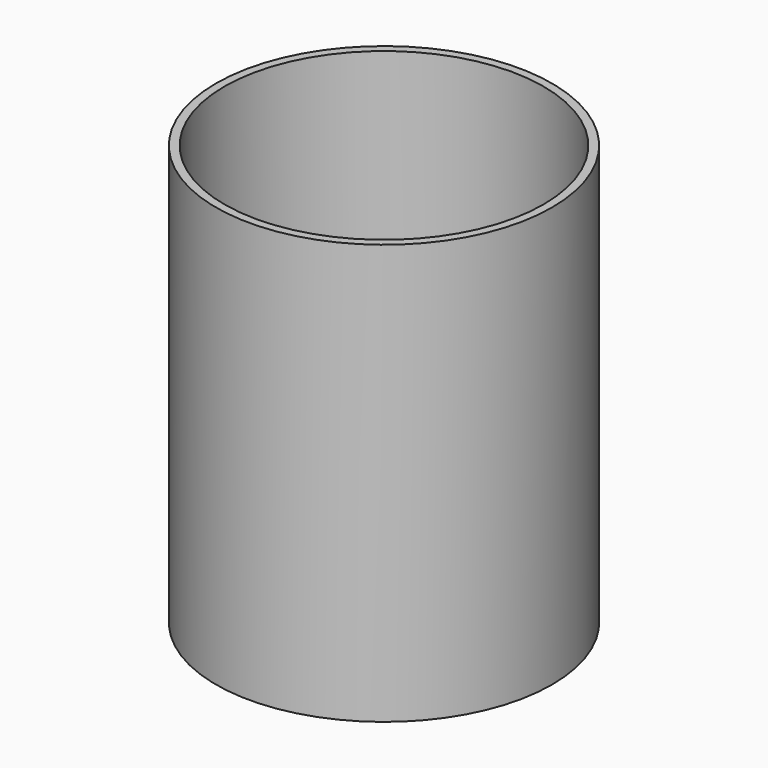
from build123d import *

# Parameters (mm, degrees)
F0_R     = 50.8
F1_DEPTH = 63.5
F2_T     = -2.54


# Not quite as in the source:
# - the program builds the solid bodies; features that only make, move or delete a surface that nothing else refers to are left out


with BuildPart() as f1:
    # F0 (on Top) → F1 (new body, symmetric)
    with BuildSketch(Plane.XY):
        Circle(F0_R)
    extrude(amount=F1_DEPTH, both=True)

    # F2
    f2_openings = [f1.faces().sort_by_distance(p)[0] for p in [
        (0, 0, 63.5),
    ]]
    offset(amount=F2_T, openings=f2_openings)


solid = f1.part
